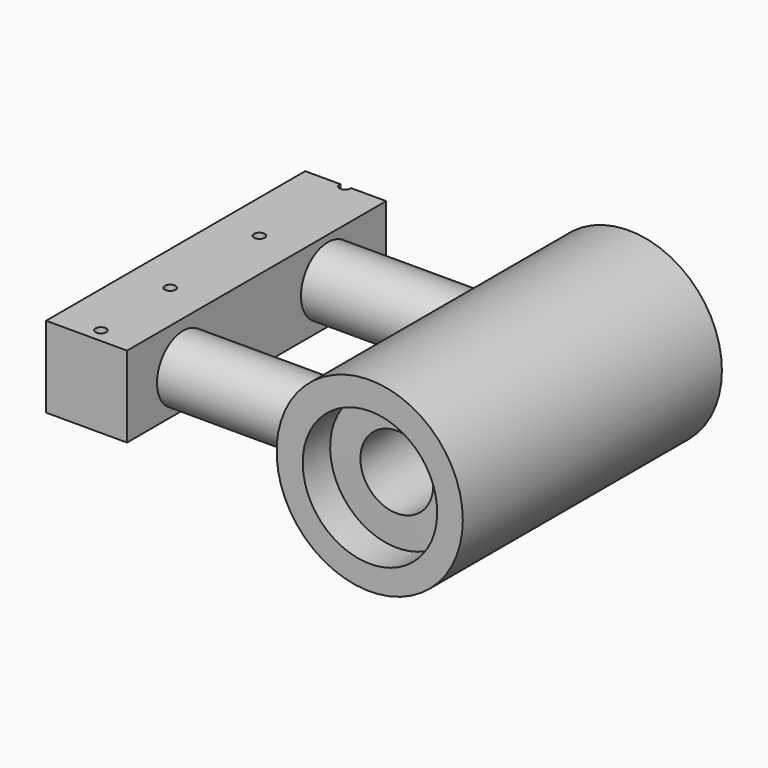
from build123d import *

# Parameters (mm, degrees)
F0_W     = 50
F0_H     = 50
F1_DEPTH = 100
F3_D     = 6.6
F4_R     = 20.2206931271
F4_R_2   = 20.8160873388
F5_DEPTH = 150
F6_R     = 57.5
F7_DEPTH = 100


with BuildPart() as f1:
    # F0 (on Front) → F1 (new body, symmetric)
    with BuildSketch(Plane.XZ):
        with Locations((25, 25)):
            Rectangle(F0_W, F0_H)
    extrude(amount=F1_DEPTH, both=True)

    # F3 (through all)
    with Locations(Plane.XY.offset(50)):
        with Locations((25, 99.4929849688), (24.9502013015, 33.496488903), (25.2753126699, -35.7510662615), (26.9008440388, -91.3441732113)):
            Hole(F3_D / 2)

    # F4 (on face) → F5 (join)
    with BuildSketch(Plane.YZ.offset(50)):
        with Locations((-56.6662251949, 23.0115242302)):
            Circle(F4_R)
        with Locations((55.072888732, 25.1332446933)):
            Circle(F4_R_2)
    extrude(amount=F5_DEPTH)

    # F6 (on Front) → F7 (join, symmetric)
    with BuildSketch(Plane.XZ):
        with Locations((199.8447626829, 25.3131054342)):
            Circle(F6_R)
    extrude(amount=F7_DEPTH, both=True)

    # F9 (on offset) → F10 (revolve, cut)
    with BuildSketch(Plane(origin=(200, 0, 0), x_dir=(0, -1, 0), z_dir=(-1, 0, 0))):
        Polygon((-105.5897921324, 24.3519060314), (100.8795276284, 24.3519060314), (101.4911159873, 24.6927142143), (105.1713102595, 25.4731605558), (104.8070022361, 65.9113094268), (79.0776162995, 65.679512918), (79.2472240509, 46.8530719335), (-62.0798177726, 45.5798540268), (-62.2608959675, 65.679512918), (-105.5897921324, 65.2891620994), align=None)
    revolve(axis=Axis((200, 2.355132252, 24.3519060314), (0, 1, 0)), mode=Mode.SUBTRACT)


solid = f1.part
